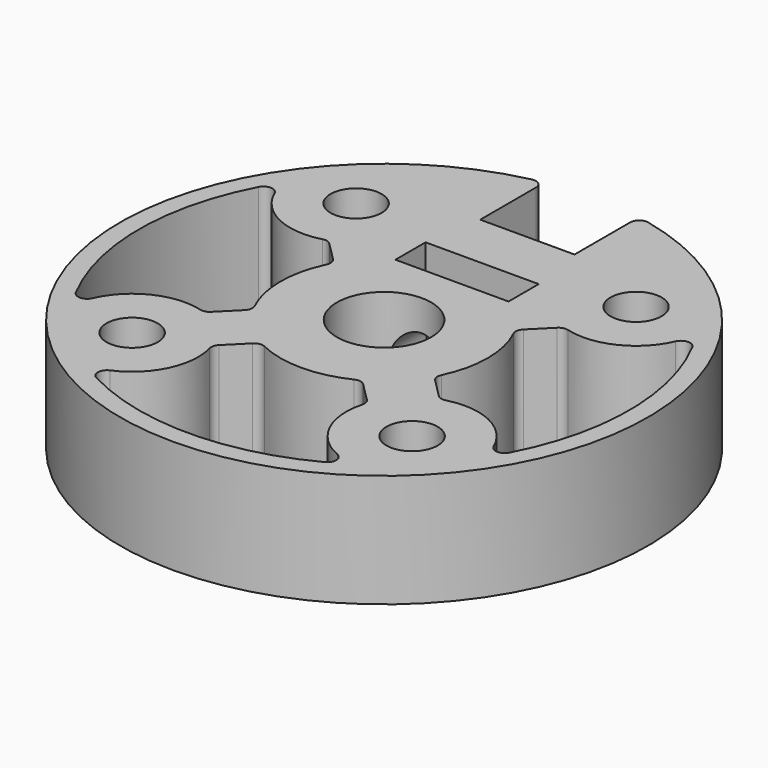
from build123d import *

# Parameters (mm, degrees)
F0_R            = 2.15265
F0_R_2          = 3.96875
F0_W            = 9.525
F0_H            = 3.175
F1_DEPTH        = 9.525
F2_R            = 2.15265
F3_REACH        = 43.3958636501
F5_R            = 3.96875
F6_DEPTH        = 3.175
F8_DEPTH        = 9.525
F8_COPIES_COUNT = 3
F8_COPIES_ANGLE = 180
F9_R            = 0.762


# Not quite as in the source:
# - a feature of the source that left no trace in its solid (it failed there, or was rolled back) is left out
# - a pattern or mirror of a feature is missing from the dataset's text; its kind, count and spacing are read off the source's solid


with BuildPart() as f1:
    # F0 (on Top) → F1 (new body)
    with BuildSketch(Plane.XY):
        with BuildLine():
            Line((3.96875, 15.08125), (-3.96875, 15.08125))
            Line((-3.96875, 15.08125), (-3.96875, 21.8677764859))
            ThreePointArc((-3.96875, 21.8677764859), (0, -22.225), (3.96875, 21.8677764859))
            Line((3.96875, 21.8677764859), (3.96875, 15.08125))
        make_face()
        with Locations((-11.7865861589, -11.7865861589)):
            Circle(F0_R, mode=Mode.SUBTRACT)
        with Locations((11.7865861589, -11.7865861589)):
            Circle(F0_R, mode=Mode.SUBTRACT)
        with Locations((-11.7865861589, 11.7865861589)):
            Circle(F0_R, mode=Mode.SUBTRACT)
        Circle(F0_R_2, mode=Mode.SUBTRACT)
        with Locations((0, 8.73125)):
            Rectangle(F0_W, F0_H, mode=Mode.SUBTRACT)
        with Locations((11.7865861589, 11.7865861589)):
            Circle(F0_R, mode=Mode.SUBTRACT)
    extrude(amount=F1_DEPTH)

    f3_end = f1.faces().sort_by_distance((-3.96875, 0, 4.7625))[0]
    # F2 (on face) → F3 (cut, up to a face of the model that its end follows)
    with BuildSketch(Plane(origin=(0, 15.08125, 0), x_dir=(-1, 0, 0), z_dir=(0, 1, 0))):
        with Locations((0, 4.7625)):
            Circle(F2_R)
    f3_long = extrude(amount=-F3_REACH, mode=Mode.PRIVATE)
    add(split(f3_long, bisect_by=f3_end, keep=Keep.ALL, mode=Mode.PRIVATE).solids().sort_by_distance((0, 15.08125, 4.7625))[0], mode=Mode.SUBTRACT)

    # F5 (on face) → F6 (cut, through all)
    with BuildSketch(Plane(origin=(0, 0, 0), x_dir=(1, 0, 0), z_dir=(0, 0, -1))):
        with Locations((11.7865861589, -11.7865861589)):
            Circle(F5_R)
        with Locations((-11.7865861589, 11.7865861589)):
            Circle(F5_R)
    extrude(amount=-F6_DEPTH, mode=Mode.SUBTRACT)

    # F7 (on face) → F8 (cut, through all)
    with BuildSketch(Plane(origin=(0, 0, 0), x_dir=(1, 0, 0), z_dir=(0, 0, -1))):
        with BuildLine():
            ThreePointArc((-17.3148424047, -11.229543123), (-14.7565267097, -7.0906978311), (-9.9206262673, -6.5530302219))
            Line((-9.9206262673, -6.5530302219), (-7.6236791242, -4.2560830788))
            ThreePointArc((-7.6236791242, -4.2560830788), (-8.73125, 0), (-7.6236791242, 4.2560830788))
            Line((-7.6236791242, 4.2560830788), (-9.9206262673, 6.5530302219))
            ThreePointArc((-9.9206262673, 6.5530302219), (-14.7565267097, 7.0906978311), (-17.3148424047, 11.229543123))
            ThreePointArc((-17.3148424047, 11.229543123), (-20.6375, 0), (-17.3148424047, -11.229543123))
        make_face()
    f8 = extrude(amount=-F8_DEPTH, mode=Mode.SUBTRACT)

    # F8_copies: F8 ×3 about axis
    f8_copies_axis = Axis((0, 0, 0), (0, 0, 1))
    for i in range(1, F8_COPIES_COUNT):
        add(f8.rotate(f8_copies_axis, i * F8_COPIES_ANGLE / (F8_COPIES_COUNT - 1)), mode=Mode.SUBTRACT)

    # F9
    f9_edges = [f1.edges().sort_by_distance(p)[0] for p in [
        (-17.314842, -11.229543, 4.7625),
        (-9.920626, -6.55303, 4.7625),
        (-7.623679, -4.256083, 4.7625),
        (-7.623679, 4.256083, 4.7625),
        (-9.920626, 6.55303, 4.7625),
        (-17.314842, 11.229543, 4.7625),
        (3.96875, 21.867776, 4.7625),
        (-3.96875, 21.867776, 4.7625),
        (11.229543, -17.314842, 4.7625),
        (-11.229543, -17.314842, 4.7625),
        (6.55303, -9.920626, 4.7625),
        (-6.55303, -9.920626, 4.7625),
        (4.256083, -7.623679, 4.7625),
        (-4.256083, -7.623679, 4.7625),
        (17.314842, 11.229543, 4.7625),
        (17.314842, -11.229543, 4.7625),
        (9.920626, 6.55303, 4.7625),
        (7.623679, 4.256083, 4.7625),
        (7.623679, -4.256083, 4.7625),
        (9.920626, -6.55303, 4.7625),
    ]]
    fillet(f9_edges, radius=F9_R)


solid = f1.part
